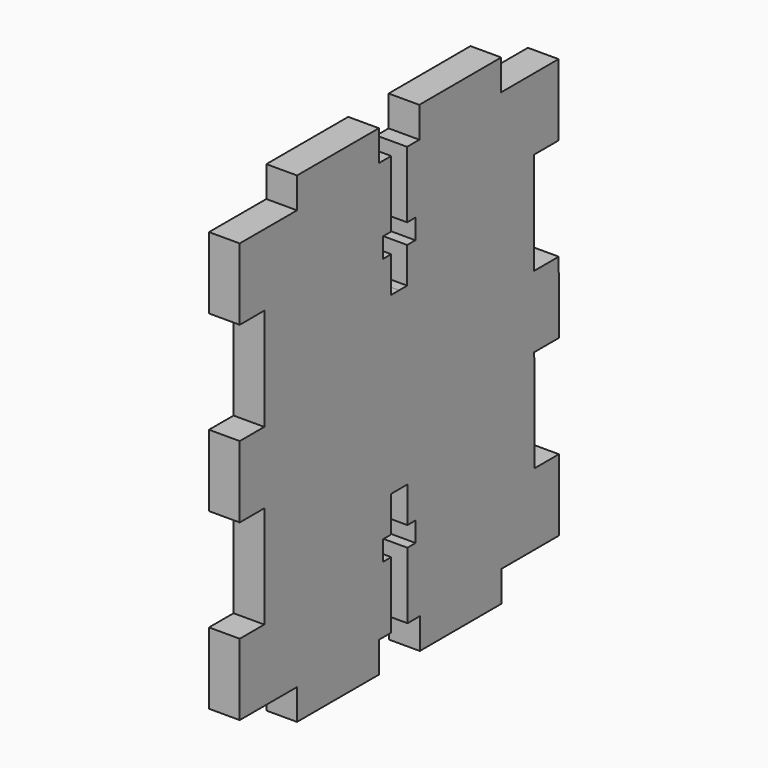
from build123d import *

# Parameters (mm, degrees)
F1_DEPTH = 3


# Not quite as in the source:
# - ends of sketch curves that miss each other by under 0.0002 mm in the source are joined


with BuildPart() as f1:
    # F0 (on Right) → F1 (new body)
    with BuildSketch(Plane.YZ):
        Polygon((-16.4821194199, 3.4866289613), (-19.4821194199, 3.4866289613), (-19.4821194199, -0.0133710387), (-19.4821194199, -3.5133710387), (-16.4821194199, -3.5133710387), (-16.4821194218, -13.5133710387), (-19.4821194199, -13.5133710387), (-19.4821194222, -20.5133710387), (-12.4821194199, -20.5133710387), (-12.4821194214, -23.5133710387), (-2.4821194199, -23.5133710387), (-2.4821194202, -20.5133710387), (-0.9821194199, -20.5133710387), (-0.98211942, -14.0133710387), (-1.9821194199, -14.0133710387), (-1.9821194199, -12.0667160037), (-0.9821194199, -12.0667160037), (-0.98211942, -8.5667160037), (-0.0066117616, -8.5667160037), (0.0178805801, -8.5667160037), (0.9933873842, -8.5654249595), (0.9979620612, -12.0654219699), (1.997962061, -12.0654219699), (2.0005064375, -14.0120753421), (1.0005064375, -14.0120753421), (1.0090022661, -20.5120697898), (2.5090009847, -20.510109214), (2.5129221366, -23.5101066514), (12.5129135944, -23.4970361461), (12.5089924443, -20.4970387087), (19.5089864635, -20.4878893549), (19.499837112, -13.4878953343), (16.4998396723, -13.4918164859), (16.4867691689, -3.4918250278), (19.4867666044, -3.4879038762), (19.4821919275, 0.0120931341), (19.4776172507, 3.5120901445), (16.4776198132, 3.5081689929), (16.4645493098, 13.508160451), (19.4645467453, 13.5120816026), (19.4553973939, 20.5120756232), (12.4554033709, 20.5029262695), (12.4514822208, 23.5029237069), (2.4514907612, 23.4898532016), (2.4554119131, 20.4898557642), (0.9554131941, 20.4878951884), (0.9639090227, 13.9879007406), (1.9639081685, 13.9892077911), (1.9639081683, 12.0425510933), (0.9664533991, 12.0412473684), (0.9710280761, 8.5412503581), (0.0178805401, 8.540004545), (-0.0289710698, 8.5399739263), (-0.9821194199, 8.5399739263), (-0.9821194199, 12.0399739263), (-1.9821194199, 12.0399739263), (-1.9821194199, 13.9866289613), (-0.9821194199, 13.9866289613), (-0.9821194199, 20.4866289613), (-2.4821194199, 20.4866289613), (-2.4821194199, 23.4866289613), (-12.4821194199, 23.4866289613), (-12.4821194199, 20.4866289613), (-19.4821194199, 20.4866289613), (-19.4821194199, 13.4866289613), (-16.4821194199, 13.4866289613), align=None)
    extrude(amount=F1_DEPTH)


solid = f1.part
